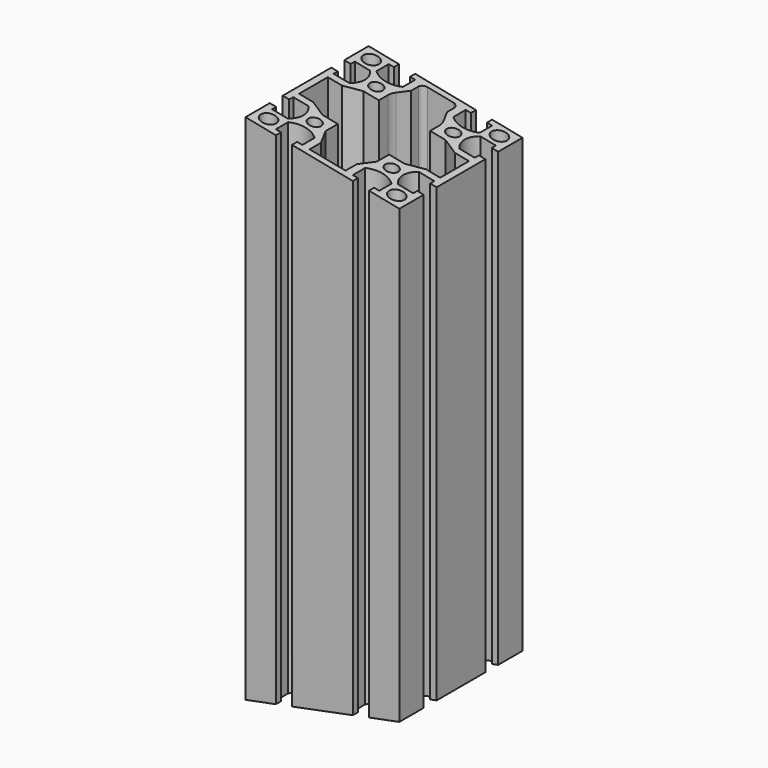
from build123d import *

# Parameters (mm, degrees)
F0_R          = 3
F0_R_2        = 2.5
F1_DEPTH      = 200
F2_R          = 2
F3_R          = 7
F6_DEPTH      = 30
F6_DEPTH_BACK = 30


# Not quite as in the source:
# - a feature names something its author has since deleted; it is built from what else it names


with BuildPart() as f1:
    # F0 (on Top) → F1 (new body)
    with BuildSketch(Plane.XY):
        with BuildLine():
            Line((18.15, -30), (30, -30))
            Line((30, -30), (30, -18.15))
            Line((30, -18.15), (27.5, -18.15))
            Line((27.5, -18.15), (27.5, -20.15))
            Line((27.5, -20.15), (21.5477069044, -20.15))
            ThreePointArc((21.5477069044, -20.15), (19.5, -15), (21.5477069044, -9.85))
            Line((21.5477069044, -9.85), (27.5, -9.85))
            Line((27.5, -9.85), (27.5, -11.85))
            Line((27.5, -11.85), (30, -11.85))
            Line((30, -11.85), (30, 11.85))
            Line((30, 11.85), (27.5, 11.85))
            Line((27.5, 11.85), (27.5, 9.85))
            Line((27.5, 9.85), (21.5477069044, 9.85))
            ThreePointArc((21.5477069044, 9.85), (19.5, 15), (21.5477069044, 20.15))
            Line((21.5477069044, 20.15), (27.5, 20.15))
            Line((27.5, 20.15), (27.5, 18.15))
            Line((27.5, 18.15), (30, 18.15))
            Line((30, 18.15), (30, 30))
            Line((30, 30), (18.15, 30))
            Line((18.15, 30), (18.15, 27.5))
            Line((18.15, 27.5), (20.15, 27.5))
            Line((20.15, 27.5), (20.15, 21.5477069044))
            ThreePointArc((20.15, 21.5477069044), (15, 19.5), (9.85, 21.5477069044))
            Line((9.85, 21.5477069044), (9.85, 27.5))
            Line((9.85, 27.5), (11.85, 27.5))
            Line((11.85, 27.5), (11.85, 30))
            Line((11.85, 30), (-11.85, 30))
            Line((-11.85, 30), (-11.85, 27.5))
            Line((-11.85, 27.5), (-9.85, 27.5))
            Line((-9.85, 27.5), (-9.85, 21.5477069044))
            ThreePointArc((-9.85, 21.5477069044), (-15, 19.5), (-20.15, 21.5477069044))
            Line((-20.15, 21.5477069044), (-20.15, 27.5))
            Line((-20.15, 27.5), (-18.15, 27.5))
            Line((-18.15, 27.5), (-18.15, 30))
            Line((-18.15, 30), (-30, 30))
            Line((-30, 30), (-30, 18.15))
            Line((-30, 18.15), (-27.5, 18.15))
            Line((-27.5, 18.15), (-27.5, 20.15))
            Line((-27.5, 20.15), (-21.5477069044, 20.15))
            ThreePointArc((-21.5477069044, 20.15), (-19.5, 15), (-21.5477069044, 9.85))
            Line((-21.5477069044, 9.85), (-27.5, 9.85))
            Line((-27.5, 9.85), (-27.5, 11.85))
            Line((-27.5, 11.85), (-30, 11.85))
            Line((-30, 11.85), (-30, -11.85))
            Line((-30, -11.85), (-27.5, -11.85))
            Line((-27.5, -11.85), (-27.5, -9.85))
            Line((-27.5, -9.85), (-21.5477069044, -9.85))
            ThreePointArc((-21.5477069044, -9.85), (-19.5, -15), (-21.5477069044, -20.15))
            Line((-21.5477069044, -20.15), (-27.5, -20.15))
            Line((-27.5, -20.15), (-27.5, -18.15))
            Line((-27.5, -18.15), (-30, -18.15))
            Line((-30, -18.15), (-30, -30))
            Line((-30, -30), (-18.15, -30))
            Line((-18.15, -30), (-18.15, -27.5))
            Line((-18.15, -27.5), (-20.15, -27.5))
            Line((-20.15, -27.5), (-20.15, -21.5477069044))
            ThreePointArc((-20.15, -21.5477069044), (-15, -19.5), (-9.85, -21.5477069044))
            Line((-9.85, -21.5477069044), (-9.85, -27.5))
            Line((-9.85, -27.5), (-11.85, -27.5))
            Line((-11.85, -27.5), (-11.85, -30))
            Line((-11.85, -30), (11.85, -30))
            Line((11.85, -30), (11.85, -27.5))
            Line((11.85, -27.5), (9.85, -27.5))
            Line((9.85, -27.5), (9.85, -21.5477069044))
            ThreePointArc((9.85, -21.5477069044), (15, -19.5), (20.15, -21.5477069044))
            Line((20.15, -21.5477069044), (20.15, -27.5))
            Line((20.15, -27.5), (18.15, -27.5))
            Line((18.15, -27.5), (18.15, -30))
        make_face()
        with Locations((-25, -25)):
            Circle(F0_R, mode=Mode.SUBTRACT)
        with Locations((-15, -15)):
            Circle(F0_R_2, mode=Mode.SUBTRACT)
        with Locations((25, -25)):
            Circle(F0_R, mode=Mode.SUBTRACT)
        with Locations((15, -15)):
            Circle(F0_R_2, mode=Mode.SUBTRACT)
        with Locations((-25, 25)):
            Circle(F0_R, mode=Mode.SUBTRACT)
        with Locations((-15, 15)):
            Circle(F0_R_2, mode=Mode.SUBTRACT)
        Polygon((-7, 22), (-7, 27.5), (0, 27.5), (7, 27.5), (7, 22), (10, 16), (10, 10), (16, 10), (22, 7), (27.5, 7), (27.5, 0), (27.5, -7), (22, -7), (16, -10), (10, -10), (10, -16), (7, -22), (7, -27.5), (0, -27.5), (-7, -27.5), (-7, -22), (-10, -16), (-10, -10), (-16, -10), (-22, -7), (-27.5, -7), (-27.5, 0), (-27.5, 7), (-22, 7), (-16, 10), (-10, 10), (-10, 16), align=None, mode=Mode.SUBTRACT)
        with Locations((15, 15)):
            Circle(F0_R_2, mode=Mode.SUBTRACT)
        with Locations((25, 25)):
            Circle(F0_R, mode=Mode.SUBTRACT)
    extrude(amount=F1_DEPTH)

    # F2
    f2_edges = [f1.edges().sort_by_distance(p)[0] for p in [
        (-7, 27.5, 100),
        (7, 27.5, 100),
    ]]
    fillet(f2_edges, radius=F2_R)

    # F3
    f3_edges = [f1.edges().sort_by_distance(p)[0] for p in [
        (-10, 16, 100),
        (10, 16, 100),
    ]]
    fillet(f3_edges, radius=F3_R)

    # F5 (on Front) → F6 (cut, two sides)
    with BuildSketch(Plane.XZ) as f6_sk:
        Polygon((161.6827257777, -158.1931300344), (124.1182914407, 30.656034207), (-30, 0), (7.5644343369, -188.8491642414), align=None)
        Polygon((119.7769204661, 170.2075181713), (153.4553825462, 339.5205806204), (3.6784620801, 369.3130624492), (-30, 200), align=None)
    extrude(amount=F6_DEPTH, mode=Mode.SUBTRACT)
    extrude(f6_sk.sketch, amount=-F6_DEPTH_BACK, mode=Mode.SUBTRACT)


solid = f1.part
